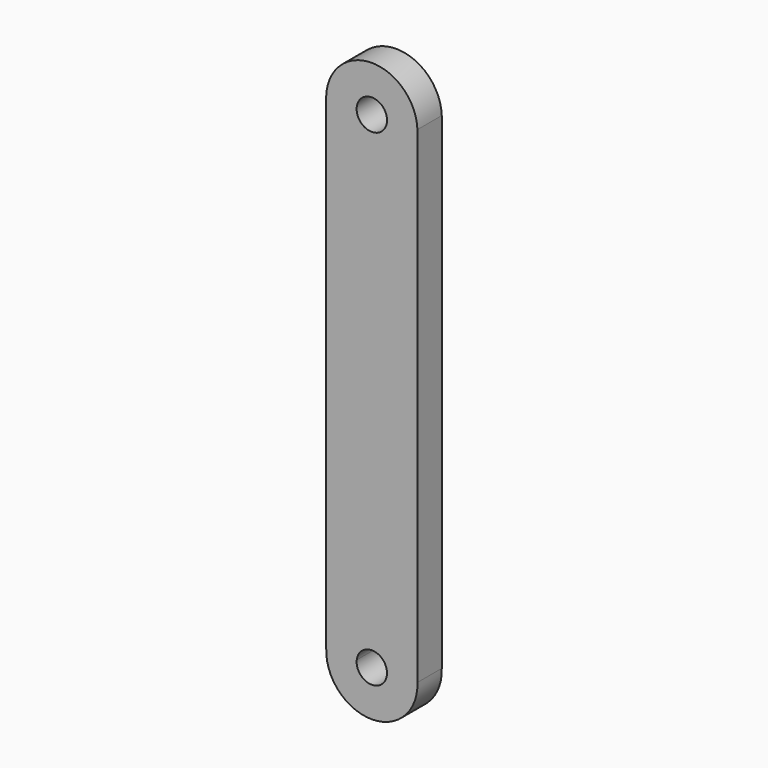
from build123d import *

# Parameters (mm, degrees)
F0_R     = 0.25
F1_DEPTH = 0.5


# Not quite as in the source:
# - a feature names something its author has since deleted; it is built from what else it names


with BuildPart() as f1:
    # F0 (on Front) → F1 (new body)
    with BuildSketch(Plane.XZ):
        with BuildLine():
            Line((-25.6771374932, 8.2580658644), (-25.1761093938, 8.2580658644))
            Line((-25.1761093938, 8.2580658644), (-25.1761093938, 16.2026529417))
            Line((-25.1761093938, 16.2026529417), (-25.1761093938, 16.2580658644))
            ThreePointArc((-25.1761093938, 16.2580658644), (-25.9255974538, 16.9803594031), (-26.6750855137, 16.2580658644))
            Line((-26.6750855137, 16.2580658644), (-26.6750855137, 16.2026529417))
            Line((-26.6750855137, 16.2026529417), (-26.6750855137, 8.2580658644))
            Line((-26.6750855137, 8.2580658644), (-26.1740574143, 8.2580658644))
            ThreePointArc((-26.1740574143, 8.2580658644), (-25.9255974538, 8.4803594031), (-25.6771374932, 8.2580658644))
        make_face()
        with Locations((-25.9255974538, 16.2303594031)):
            Circle(F0_R, mode=Mode.SUBTRACT)
        with BuildLine():
            ThreePointArc((-26.6750855137, 8.2580658644), (-25.9255974538, 7.4803594031), (-25.1761093938, 8.2580658644))
            Line((-25.1761093938, 8.2580658644), (-25.6771374932, 8.2580658644))
            ThreePointArc((-25.6771374932, 8.2580658644), (-25.6759827606, 8.2442340177), (-25.6755974538, 8.2303594031))
            ThreePointArc((-25.6755974538, 8.2303594031), (-25.9394720684, 7.9807447099), (-26.1740574143, 8.2580658644))
            Line((-26.1740574143, 8.2580658644), (-26.6750855137, 8.2580658644))
        make_face()
    extrude(amount=F1_DEPTH)


solid = f1.part
